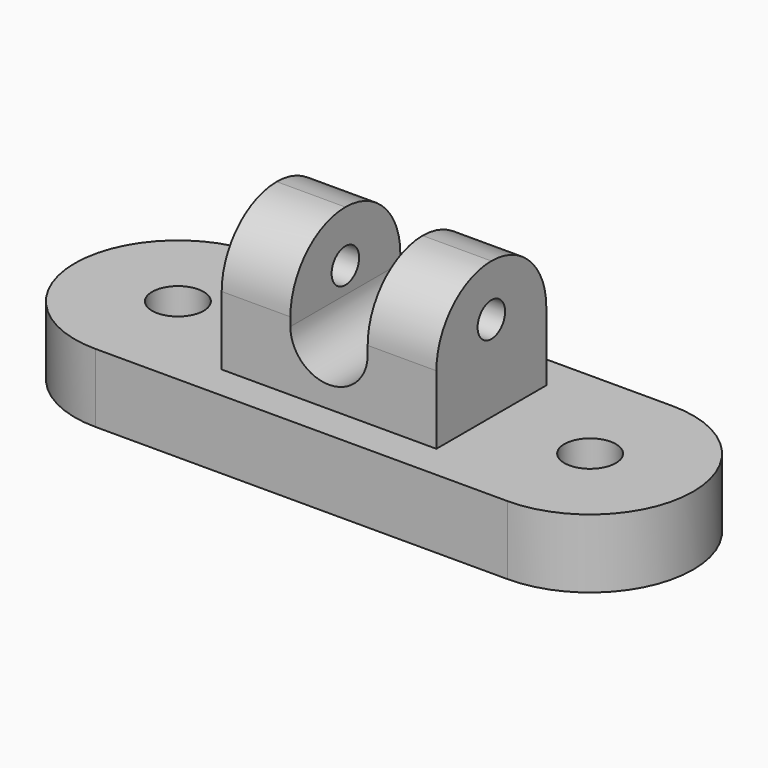
from build123d import *

# Parameters (mm, degrees)
F1_DEPTH  = 25.4
F2_W      = 79.375
F2_H      = 50.8
F3_DEPTH  = 50.8
F5_DEPTH  = 63.501
F6_R      = 25.39999
F7_R      = 6.35
F8_DEPTH  = 127
F9_R      = 9.525
F10_DEPTH = 25.401


# Not quite as in the source:
# - a fillet or chamfer is up to 0.001 mm smaller than in the source, because OpenCascade refuses the exact size


with BuildPart() as f1:
    # F0 (on Top) → F1 (new body)
    with BuildSketch(Plane.XY):
        with BuildLine():
            ThreePointArc((76.2, -38.1), (114.3, 0), (76.2, 38.1))
            Line((76.2, 38.1), (-76.2, 38.1))
            ThreePointArc((-76.2, 38.1), (-114.3, 0), (-76.2, -38.1))
            Line((-76.2, -38.1), (76.2, -38.1))
        make_face()
    extrude(amount=F1_DEPTH)

    # F2 (on face) → F3 (join)
    with BuildSketch(Plane.XY.offset(25.4)):
        Rectangle(F2_W, F2_H)
    extrude(amount=F3_DEPTH)

    # F4 (on face) → F5 (cut, through all)
    with BuildSketch(Plane.XZ.offset(25.4)):
        with BuildLine():
            Line((14.2875, 76.2), (-14.2875, 76.2))
            Line((-14.2875, 76.2), (-14.2875, 47.625))
            ThreePointArc((-14.2875, 47.625), (0, 33.3375), (14.2875, 47.625))
            Line((14.2875, 47.625), (14.2875, 76.2))
        make_face()
    extrude(amount=-F5_DEPTH, mode=Mode.SUBTRACT)

    # F6 (radius 25.4 in the source; OpenCascade refuses exactly that, so slightly less here)
    f6_edges = [f1.edges().sort_by_distance(p)[0] for p in [
        (-26.9875, -25.4, 76.2),
        (-26.9875, 25.4, 76.2),
        (26.9875, -25.4, 76.2),
        (26.9875, 25.4, 76.2),
    ]]
    fillet(f6_edges, radius=F6_R)

    # F7 (on face) → F8 (cut)
    with BuildSketch(Plane(origin=(-39.6875, 0, 0), x_dir=(0, -1, 0), z_dir=(-1, 0, 0))):
        with Locations((0, 57.15)):
            Circle(F7_R)
    extrude(amount=-F8_DEPTH, mode=Mode.SUBTRACT)

    # F9 (on face) → F10 (cut, through all)
    with BuildSketch(Plane.XY.offset(25.4)):
        with Locations((-76.2, 0)):
            Circle(F9_R)
        with Locations((76.2, 0)):
            Circle(F9_R)
    extrude(amount=-F10_DEPTH, mode=Mode.SUBTRACT)


solid = f1.part
